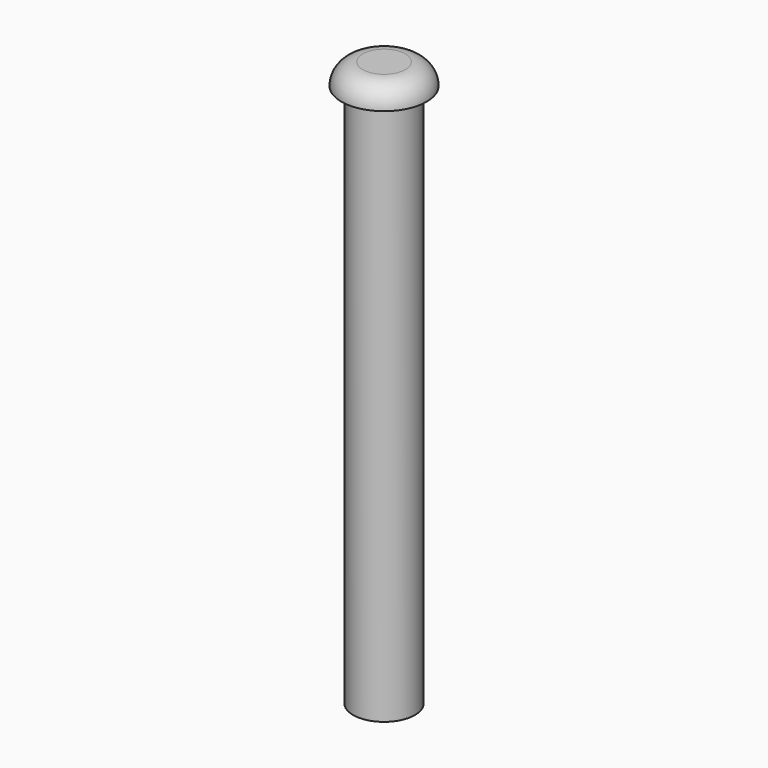
from build123d import *

# Parameters (mm, degrees)
F0_R     = 3.683
F1_DEPTH = 64.77
F2_R     = 5.08
F3_DEPTH = 2.54
F4_R     = 2.53999
F5_R     = 2.54
F6_DEPTH = 12.7


# Not quite as in the source:
# - a fillet or chamfer is up to 0.001 mm smaller than in the source, because OpenCascade refuses the exact size


with BuildPart() as f1:
    # F0 (on Top) → F1 (new body)
    with BuildSketch(Plane.XY):
        Circle(F0_R)
    extrude(amount=F1_DEPTH)

    # F2 (on face) → F3 (join)
    with BuildSketch(Plane.XY.offset(64.77)):
        Circle(F2_R)
    extrude(amount=F3_DEPTH)

    # F4 (radius 2.54 in the source; OpenCascade refuses exactly that, so slightly less here)
    f4_edges = [f1.edges().sort_by_distance(p)[0] for p in [
        (-5.08, 0, 67.31),
    ]]
    fillet(f4_edges, radius=F4_R)

    # F5 (on face) → F6 (cut)
    with BuildSketch(Plane(origin=(0, 0, 0), x_dir=(1, 0, 0), z_dir=(0, 0, -1))):
        Circle(F5_R)
    extrude(amount=-F6_DEPTH, mode=Mode.SUBTRACT)


solid = f1.part
